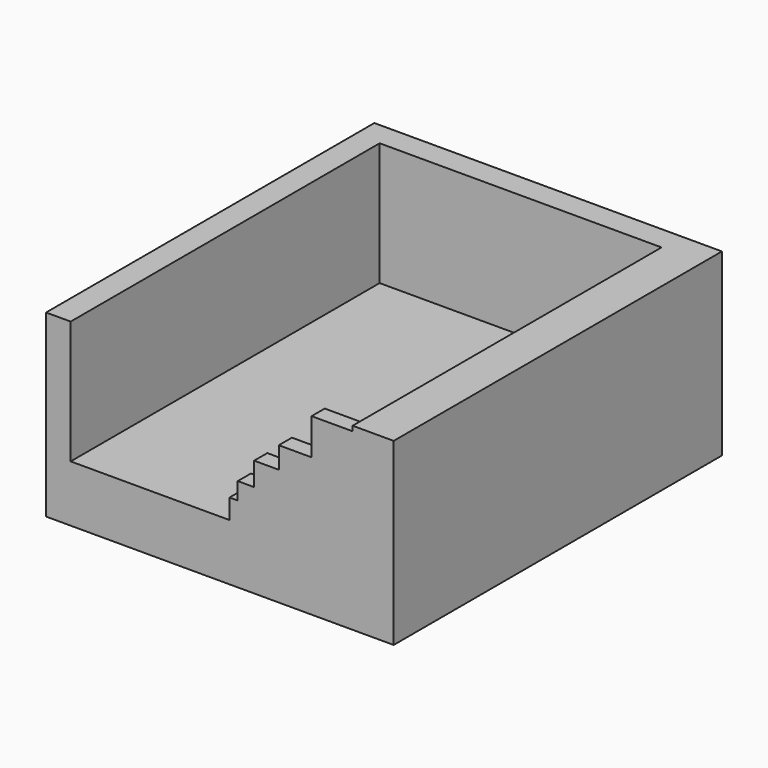
from build123d import *

# Parameters (mm, degrees)
F0_W     = 7.62
F0_H     = 38.1
F0_W_2   = 12.7
F1_DEPTH = 127
F2_W     = 87.2650571496
F2_H     = 7.4778180569
F3_DEPTH = 38.1
F5_W     = 2.54
F5_H     = 6.1494747632
F6_DEPTH = 5.08


with BuildPart() as f1:
    # F0 (on Front) → F1 (new body)
    with BuildSketch(Plane.XZ):
        Polygon((-64.6448548068, -3.3340927702), (-64.6448548068, -20.8513359327), (42.9402023428, -20.8513359327), (42.9402023428, -3.3340927702), (30.2402023428, -3.3340927702), (-57.0248548068, -3.3340927702), align=None)
        with Locations((-60.8348548068, 15.7159072298)):
            Rectangle(F0_W, F0_H)
        with Locations((36.5902023428, 15.7159072298)):
            Rectangle(F0_W_2, F0_H)
    extrude(amount=F1_DEPTH)

    # F2 (on face) → F3 (join)
    with BuildSketch(Plane.XY.offset(-3.3340927702)):
        with Locations((-13.392326232, -3.7389090285)):
            Rectangle(F2_W, F2_H)
    extrude(amount=F3_DEPTH)

    # F5 (on face) → F6 (join)
    with BuildSketch(Plane.XZ.offset(127)):
        Polygon((30.2402023428, -3.3340927702), (30.2402023428, 33.2476731723), (17.5402023428, 33.2476731723), (17.5402023428, 22.0181959489), (17.5402023428, -3.3340927702), align=None)
        Polygon((17.5402023428, -3.3340927702), (17.5402023428, 22.0181959489), (7.3802023428, 22.0181959489), (7.3802023428, 15.3339850341), (7.3802023428, -3.3340927702), align=None)
        Polygon((-0.2397976572, -3.3340927702), (7.3802023428, -3.3340927702), (7.3802023428, 15.3339850341), (-0.2397976572, 15.3339850341), (-0.2397976572, 8.1150363277), align=None)
        Polygon((-5.3197976572, -3.3340927702), (-0.2397976572, -3.3340927702), (-0.2397976572, 8.1150363277), (-5.3197976572, 8.1150363277), (-5.3197976572, 2.8153819931), align=None)
        with Locations((-6.5897976572, -0.2593553885)):
            Rectangle(F5_W, F5_H)
    extrude(amount=-F6_DEPTH)


solid = f1.part
